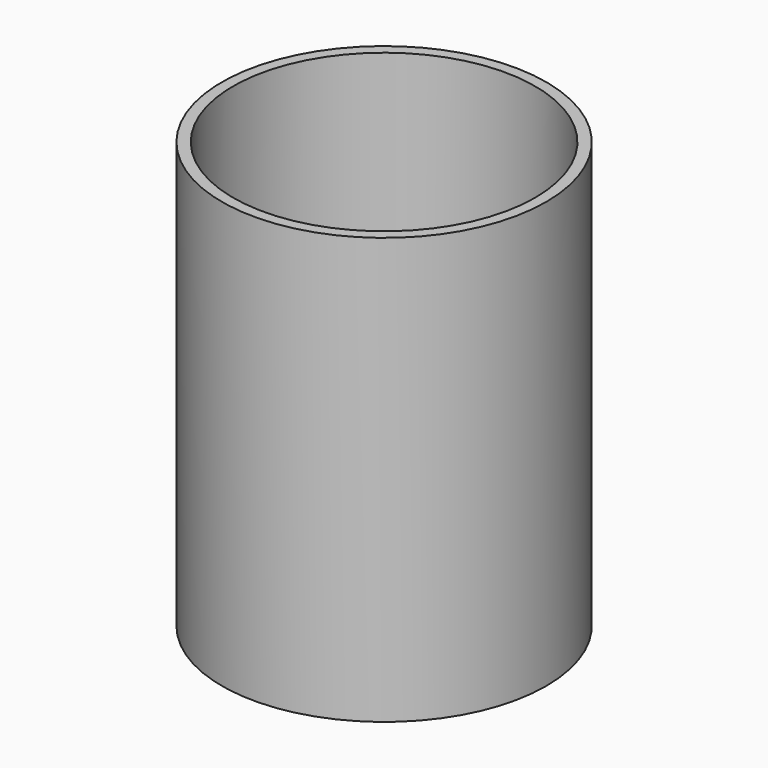
from build123d import *

# Parameters (mm, degrees)
F2_R      = 14.5
F2_R_2    = 13.5
F8_DEPTH  = 38.1
F10_R     = 13.5900846428
F10_R_2   = 12
F11_DEPTH = 5
F12_R     = 1


# Not quite as in the source:
# - the program builds the solid bodies; features that only make, move or delete a surface that nothing else refers to are left out


with BuildPart() as f8:
    # F2 (on offset) → F8 (new body)
    with BuildSketch(Plane.XY.offset(76.2)):
        Circle(F2_R)
        Circle(F2_R_2, mode=Mode.SUBTRACT)
    extrude(amount=F8_DEPTH)


with BuildPart() as f11:
    # F10 (on offset) → F11 (new body)
    with BuildSketch(Plane.XY.offset(76.2)):
        Circle(F10_R)
        Circle(F10_R_2, mode=Mode.SUBTRACT)
    extrude(amount=F11_DEPTH)

    # F12
    f12_edges = [f11.edges().sort_by_distance(p)[0] for p in [
        (-13.590085, 0, 76.2),
        (-13.590085, 0, 81.2),
    ]]
    fillet(f12_edges, radius=F12_R)


solid = Compound([f8.part, f11.part])
